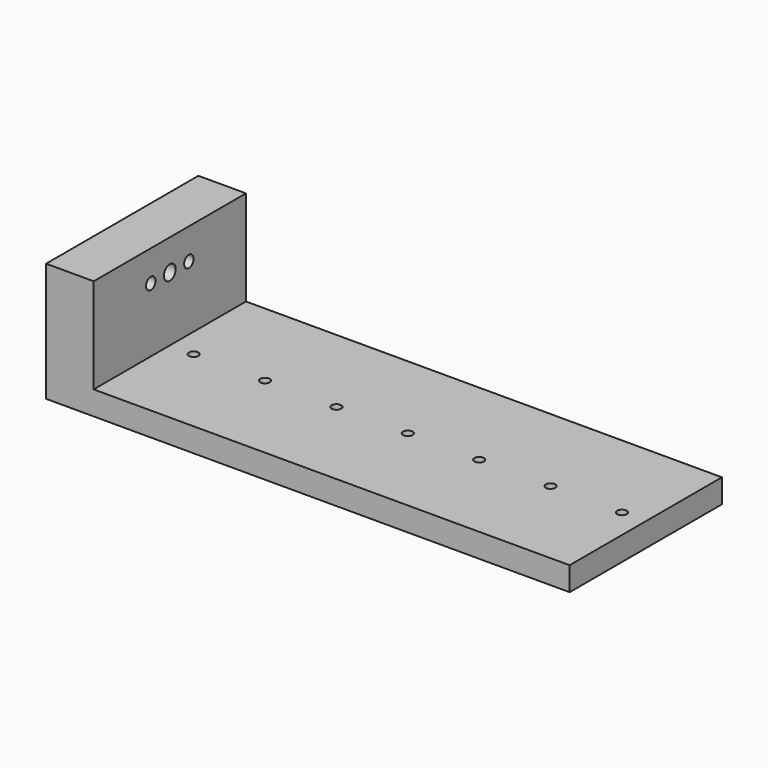
from build123d import *

# Parameters (mm, degrees)
F1_DEPTH = 80
F2_R     = 2
F3_DEPTH = 25
F4_R     = 2.5
F5_DEPTH = 22
F4_R_2   = 3.1
F6_DEPTH = 5


# Not quite as in the source:
# - a feature names something its author has since deleted; it is built from what else it names


with BuildPart() as f1:
    # F0 (on Front) → F1 (new body)
    with BuildSketch(Plane.XZ):
        Polygon((-110, -25), (110, -25), (110, -15), (-90, -15), (-90, 25), (-110, 25), align=None)
    extrude(amount=F1_DEPTH)

    # F2 (on face) → F3 (cut)
    with BuildSketch(Plane.XY.offset(-15)):
        with Locations((-80, -40)):
            Circle(F2_R)
        with Locations((-50, -40)):
            Circle(F2_R)
        with Locations((-20, -40)):
            Circle(F2_R)
        with Locations((10, -40)):
            Circle(F2_R)
        with Locations((40, -40)):
            Circle(F2_R)
        with Locations((70, -40)):
            Circle(F2_R)
        with Locations((100, -40)):
            Circle(F2_R)
    extrude(amount=-F3_DEPTH, mode=Mode.SUBTRACT)

    # F4 (on face) → F5 (cut)
    with BuildSketch(Plane.YZ.offset(-90)):
        with Locations((-50, 12)):
            Circle(F4_R)
        with Locations((-30, 12)):
            Circle(F4_R)
    extrude(amount=-F5_DEPTH, mode=Mode.SUBTRACT)

    # F4 (on face) → F6 (cut)
    with BuildSketch(Plane.YZ.offset(-90)):
        with Locations((-40, 12)):
            Circle(F4_R_2)
    extrude(amount=-F6_DEPTH, mode=Mode.SUBTRACT)


solid = f1.part
